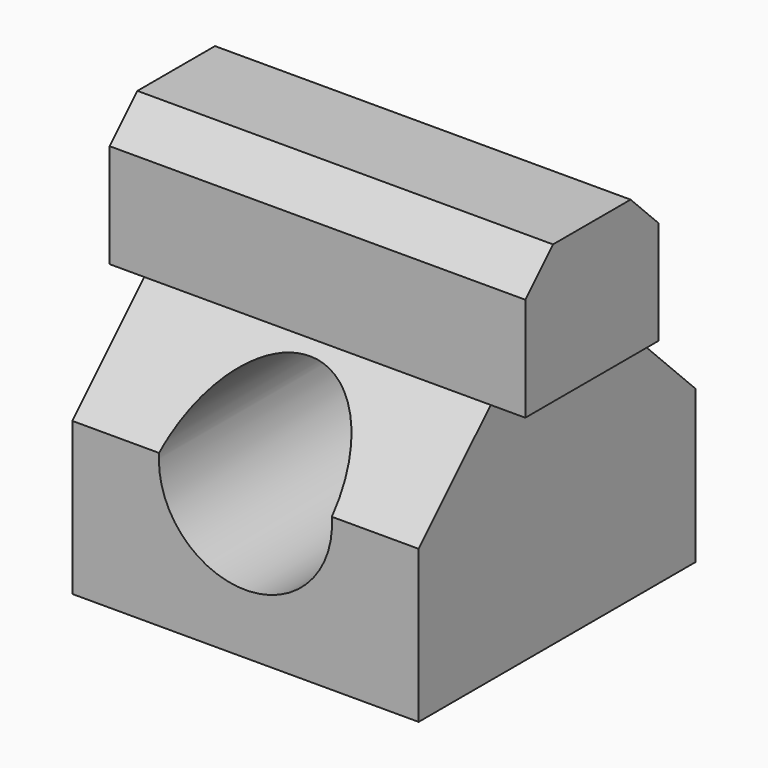
from build123d import *

# Parameters (mm, degrees)
F0_W        = 50
F0_H        = 50
F1_DEPTH    = 35
F3_D        = 25
F4_T1_DEPTH = 116.8637576871
F5_T1_DEPTH = 116.8637576871
F6_DEPTH    = 20
F7_T1_DEPTH = 75.7168298797
F10_DEPTH   = 5
F12_DEPTH   = 5


# Not quite as in the source:
# - a fillet or chamfer that OpenCascade refuses, or shapes differently, is made with other operations: its cross-section is extruded or revolved along the edge and cut away or added
# - two fillets or chamfers of one size are made in one step


with BuildPart() as f1:
    # F0 (on Top) → F1 (new body)
    with BuildSketch(Plane.XY):
        with Locations((25, 25)):
            Rectangle(F0_W, F0_H)
    extrude(amount=F1_DEPTH)

    # F3 (through all)
    with Locations(Plane.XZ):
        with Locations((25, 21.1336053908)):
            Hole(F3_D / 2)

    # F4: chamfer of 13 on 1 edges, made by hand

    # F4_s2 → F4_t1 (cut)
    with BuildSketch(Plane.YZ.offset(-33.4318788436)):
        Polygon((0, 22), (13, 35), (0, 35), align=None)
    extrude(amount=F4_T1_DEPTH, mode=Mode.SUBTRACT)

    # F5: chamfer of 13 on 1 edges, made by hand

    # F5_s2 → F5_t1 (cut)
    with BuildSketch(Plane.YZ.offset(-33.4318788436)):
        Polygon((37, 35), (50, 22), (50, 35), align=None)
    extrude(amount=F5_T1_DEPTH, mode=Mode.SUBTRACT)

    # F6 (add): a face of the model
    f6_faces = [f1.faces().sort_by_distance(p)[0] for p in [
        (25, 25, 35),
    ]]
    extrude(f6_faces, amount=F6_DEPTH)

    # F7: chamfer of 5 on 4 edges, made by hand

    # F7_s2 → F7_t1 (cut)
    with BuildSketch(Plane.YZ.offset(-12.8584149398)):
        Polygon((13, 50), (18, 55), (13, 55), align=None)
        Polygon((37, 50), (32, 55), (37, 55), align=None)
    extrude(amount=F7_T1_DEPTH, mode=Mode.SUBTRACT)

    # F9 (on face) → F10 (join)
    with BuildSketch(Plane.YZ.offset(50)):
        Polygon((13, 50), (13, 35), (37, 35), (37, 50), (32, 55), (18, 55), align=None)
    extrude(amount=F10_DEPTH)

    # F11 (on face) → F12 (join)
    with BuildSketch(Plane(origin=(0, 0, 0), x_dir=(0, -1, 0), z_dir=(-1, 0, 0))):
        Polygon((-37, 50), (-37, 35), (-13, 35), (-13, 50), (-18, 55), (-32, 55), align=None)
    extrude(amount=F12_DEPTH)


solid = f1.part
